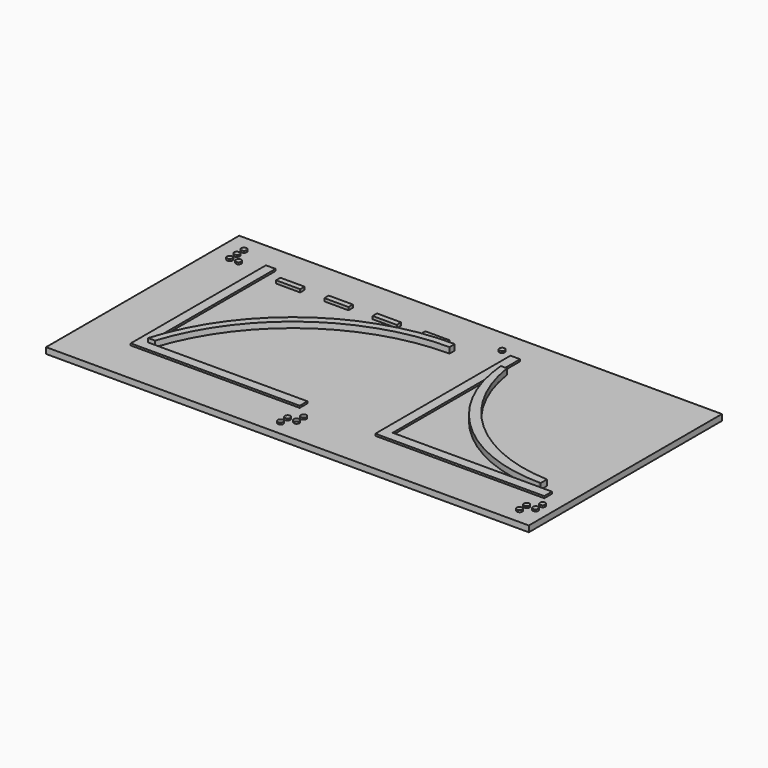
from build123d import *

# Parameters (mm, degrees)
F0_W     = 127
F0_H     = 63.5
F1_DEPTH = 1.5875
F3_DEPTH = 0.508
F4_W     = 6.35
F4_H     = 1.4422908425
F5_DEPTH = 0.762
F7_DEPTH = 1.524
F8_R     = 0.7239
F9_DEPTH = 0.4826


# Not quite as in the source:
# - a feature names something its author has since deleted; it is built from what else it names


with BuildPart() as f1:
    # F0 (on Top) → F1 (new body)
    with BuildSketch(Plane.XY):
        with Locations((63.5, 31.75)):
            Rectangle(F0_W, F0_H)
    extrude(amount=F1_DEPTH)

    # F2 (on face) → F3 (join)
    with BuildSketch(Plane.XY.offset(1.5875)):
        Polygon((15.6702585518, 55.88), (13.1302586973, 55.88), (13.1302586973, 11.43), (57.5802586973, 11.43), (57.5802586973, 13.9699998546), (55.0402588427, 13.9699998546), (15.6702585518, 13.9699998546), (15.6702585518, 53.3400001454), align=None)
        Polygon((80.009996891, 55.88), (77.47, 55.88), (77.47, 11.43), (121.92, 11.43), (121.92, 13.969996891), (119.380003109, 13.969996891), (80.009996891, 13.969996891), (80.009996891, 53.340003109), align=None)
    extrude(amount=F3_DEPTH)

    # F4 (on face) → F5 (join)
    with BuildSketch(Plane.XY.offset(1.5875)):
        with Locations((60.5010928452, 52.3195564747)):
            Rectangle(F4_W, F4_H)
        with Locations((47.8010928452, 52.3195564747)):
            Rectangle(F4_W, F4_H)
        with Locations((35.1010928452, 52.3195564747)):
            Rectangle(F4_W, F4_H)
        with Locations((22.4010928452, 52.3195564747)):
            Rectangle(F4_W, F4_H)
    extrude(amount=F5_DEPTH)

    # F8 (on face) → F9 (join)
    with BuildSketch(Plane.XY.offset(1.5875)):
        with Locations((5.095858312, 58.6940389134)):
            Circle(F8_R)
        with Locations((5.0986883188, 56.357240627)):
            Circle(F8_R)
        with Locations((5.1015183256, 54.0204423407)):
            Circle(F8_R)
        with Locations((7.4383183256, 54.0204423407)):
            Circle(F8_R)
        with Locations((58.7118677795, 3.7288046442)):
            Circle(F8_R)
        with Locations((58.7090377727, 6.0656029305)):
            Circle(F8_R)
        with Locations((61.0458377727, 6.0656029305)):
            Circle(F8_R)
        with Locations((61.043007766, 8.4024012169)):
            Circle(F8_R)
        with Locations((74.3398889899, 57.0295006037)):
            Circle(F8_R)
        with Locations((121.4120164514, 3.9590690285)):
            Circle(F8_R)
        with Locations((121.4091864446, 6.2958673148)):
            Circle(F8_R)
        with Locations((123.7431564378, 8.6326656012)):
            Circle(F8_R)
        with Locations((123.7459864446, 6.2958673148)):
            Circle(F8_R)
    extrude(amount=F9_DEPTH)


with BuildPart() as f7:
    # F6 (on face) → F7 (new body)
    with BuildSketch(Plane.XY.offset(1.5875)):
        with BuildLine():
            Line((81.6376388848, 49.51094836), (80.009996891, 49.51094836))
            ThreePointArc((80.009996891, 49.51094836), (92.3901641709, 24.2680426815), (118.5516450515, 13.969996891))
            Line((118.5516450515, 13.969996891), (118.9480349422, 13.969996891))
            Line((118.9480349422, 13.969996891), (118.9480349422, 16.0472020507))
            ThreePointArc((118.9480349422, 16.0472020507), (94.289218877, 26.0853426911), (81.6376388848, 49.51094836))
        make_face()
    extrude(amount=F7_DEPTH)


with BuildPart() as f7b:
    # F6 (on face) → F7, piece 2 (new body)
    with BuildSketch(Plane.XY.offset(1.5875)):
        with BuildLine():
            Line((66.5227174759, 49.51094836), (66.5227174759, 51.2246415019))
            ThreePointArc((66.5227174759, 51.2246415019), (34.8358116044, 41.1431226473), (15.6702585518, 13.9699998546))
            Line((15.6702585518, 13.9699998546), (17.489053309, 13.9699998546))
            ThreePointArc((17.489053309, 13.9699998546), (36.2136378026, 39.7316824187), (66.5227174759, 49.51094836))
        make_face()
    extrude(amount=F7_DEPTH)


solid = Compound([f1.part, f7.part, f7b.part])
